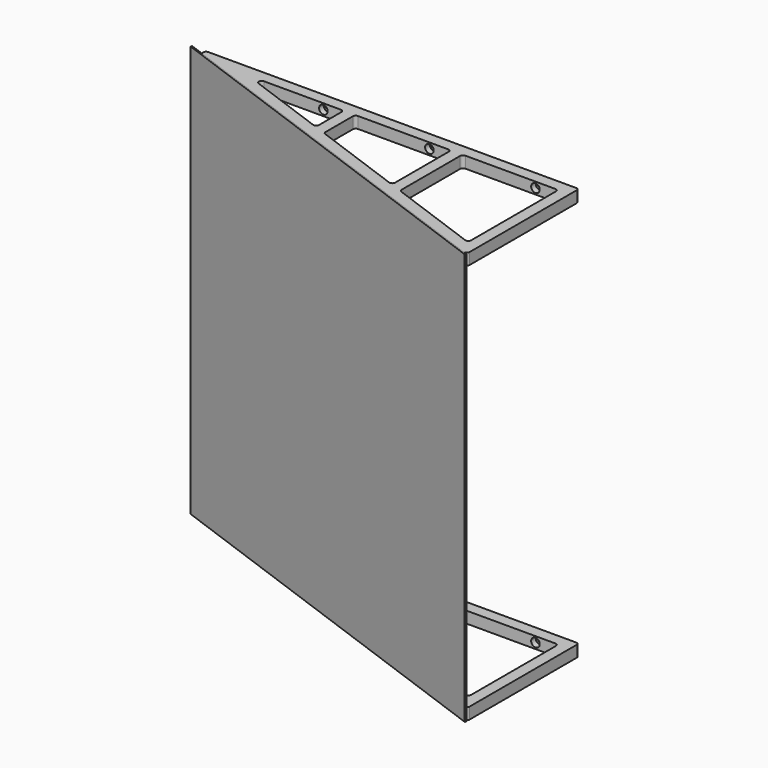
from build123d import *

# Parameters (mm, degrees)
F4_DEPTH  = 25.4
F6_DEPTH  = 25.401
F7_R      = 6.35
F8_R      = 6.35
F10_R     = 9.525
F10_R_2   = 4.7625
F11_DEPTH = 38.1
F12_DEPTH = 12.701
F14_W     = 914.4
F14_H     = 914.4
F15_DEPTH = 3.175


with BuildPart() as f4:
    # F3 (on offset) → F4 (new body)
    with BuildSketch(Plane.XY.offset(457.2)):
        Polygon((0, 0), (859.2549324466, -312.743219057), (859.2549324466, 0), align=None)
    extrude(amount=-F4_DEPTH)

    # F5 (on face) → F6 (cut, through all)
    with BuildSketch(Plane.XY.offset(457.2)):
        Polygon((144.0505582183, -25.4), (357.0520162944, -102.926190595), (357.0520162944, -25.4), align=None)
        Polygon((382.4520162944, -112.1710345454), (595.4534743705, -189.6972251404), (595.4534743705, -25.4), (382.4520162944, -25.4), align=None)
        Polygon((620.8534743705, -198.9420690907), (833.8549324466, -276.4682596857), (833.8549324466, -25.4), (620.8534743705, -25.4), align=None)
    extrude(amount=-F6_DEPTH, mode=Mode.SUBTRACT)

    # F7
    f7_edges = [f4.edges().sort_by_distance(p)[0] for p in [
        (0, 0, 444.5),
        (859.254932, -312.743219, 444.5),
        (859.254932, 0, 444.5),
    ]]
    fillet(f7_edges, radius=F7_R)

    # F8
    f8_edges = [f4.edges().sort_by_distance(p)[0] for p in [
        (144.050558, -25.4, 444.5),
        (382.452016, -112.171035, 444.5),
        (382.452016, -25.4, 444.5),
        (620.853474, -25.4, 444.5),
        (620.853474, -198.942069, 444.5),
        (357.052016, -25.4, 444.5),
        (595.453474, -25.4, 444.5),
        (833.854932, -25.4, 444.5),
        (357.052016, -102.926191, 444.5),
        (595.453474, -189.697225, 444.5),
        (833.854932, -276.46826, 444.5),
    ]]
    fillet(f8_edges, radius=F8_R)

    # F10 (on offset) → F11 (cut)
    with BuildSketch(Plane.XZ.offset(12.7)):
        with Locations((76.2, 444.5)):
            Circle(F10_R)
        with Locations((76.2, 444.5)):
            Circle(F10_R_2, mode=Mode.SUBTRACT)
        with Locations((311.8183108155, 444.5)):
            Circle(F10_R)
        with Locations((311.8183108155, 444.5)):
            Circle(F10_R_2, mode=Mode.SUBTRACT)
        with Locations((547.4366216311, 444.5)):
            Circle(F10_R)
        with Locations((547.4366216311, 444.5)):
            Circle(F10_R_2, mode=Mode.SUBTRACT)
        with Locations((783.0549324466, 444.5)):
            Circle(F10_R)
        with Locations((783.0549324466, 444.5)):
            Circle(F10_R_2, mode=Mode.SUBTRACT)
        with Locations((76.2, 444.5)):
            Circle(F10_R_2)
        with Locations((311.8183108155, 444.5)):
            Circle(F10_R_2)
        with Locations((547.4366216311, 444.5)):
            Circle(F10_R_2)
        with Locations((783.0549324466, 444.5)):
            Circle(F10_R_2)
    extrude(amount=F11_DEPTH, mode=Mode.SUBTRACT)

    # F10 (on offset) → F12 (cut, through all)
    with BuildSketch(Plane.XZ.offset(12.7)):
        with Locations((76.2, 444.5)):
            Circle(F10_R_2)
        with Locations((311.8183108155, 444.5)):
            Circle(F10_R_2)
        with Locations((547.4366216311, 444.5)):
            Circle(F10_R_2)
        with Locations((783.0549324466, 444.5)):
            Circle(F10_R_2)
    extrude(amount=-F12_DEPTH, mode=Mode.SUBTRACT)


with BuildPart() as f13_1:
    # F13: instance of F4
    add(f4.part.mirror(Plane.XY))


with BuildPart() as f15:
    # F14 (on face) → F15 (new body)
    with BuildSketch(Plane(origin=(0, 0, 0), x_dir=(0.9396926208, -0.3420201433, 0), z_dir=(-0.3420201433, -0.9396926208, 0))):
        with Locations((457.2, 0)):
            Rectangle(F14_W, F14_H)
    extrude(amount=F15_DEPTH)


solid = Compound([f4.part, f13_1.part, f15.part])
